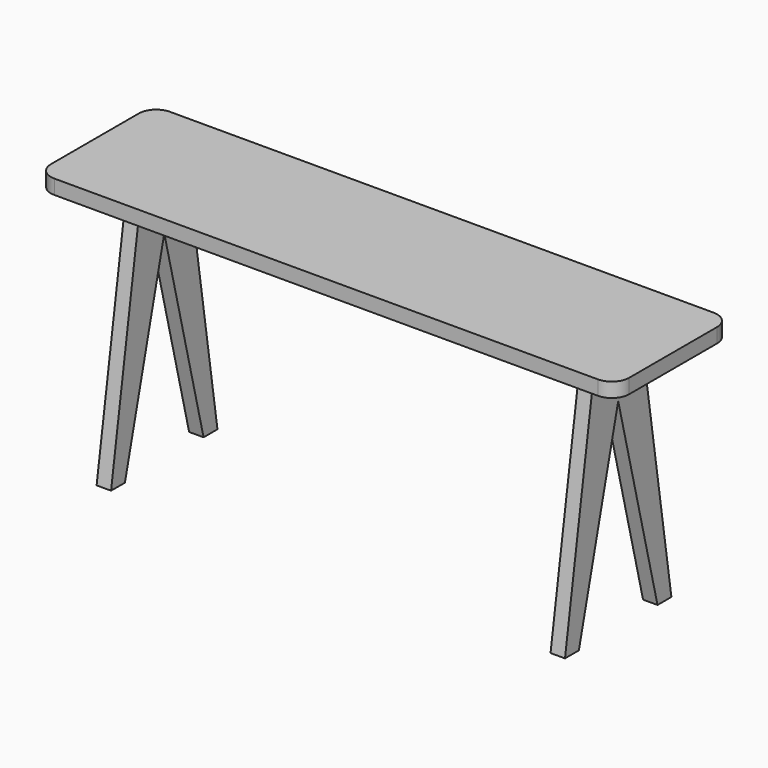
from build123d import *

# Parameters (mm, degrees)
F0_W     = 1000
F0_H     = 250
F1_DEPTH = 25
F2_W     = 380
F2_H     = 70
F3_DEPTH = 12.5
F5_START = 380
F5_DEPTH = 25
F6_START = -380
F6_DEPTH = 25
F7_R     = 30


with BuildPart() as f1:
    # F0 (on Top) → F1 (new body)
    with BuildSketch(Plane.XY):
        Rectangle(F0_W, F0_H)
    extrude(amount=F1_DEPTH)

    # F2 (on Front) → F3 (join, symmetric)
    with BuildSketch(Plane.XZ):
        with Locations((-190, -35)):
            Rectangle(F2_W, F2_H)
        with Locations((190, -35)):
            Rectangle(F2_W, F2_H)
    extrude(amount=F3_DEPTH, both=True)

    # F4 (on Right) → F5 (join)
    with BuildSketch(Plane.YZ.offset(F5_START)):
        Polygon((50, 0), (0, 0), (0, -80), (85, -425), (115, -425), align=None)
        Polygon((0, -80), (0, 0), (-50, 0), (-115, -425), (-85, -425), align=None)
    extrude(amount=F5_DEPTH)

    # F4 (on Right) → F6 (join)
    with BuildSketch(Plane.YZ.offset(F6_START)):
        Polygon((0, -80), (0, 0), (-50, 0), (-115, -425), (-85, -425), align=None)
        Polygon((50, 0), (0, 0), (0, -80), (85, -425), (115, -425), align=None)
    extrude(amount=-F6_DEPTH)

    # F7
    f7_edges = [f1.edges().sort_by_distance(p)[0] for p in [
        (500, 125, 12.5),
        (500, -125, 12.5),
        (-500, 125, 12.5),
        (-500, -125, 12.5),
    ]]
    fillet(f7_edges, radius=F7_R)


solid = f1.part
